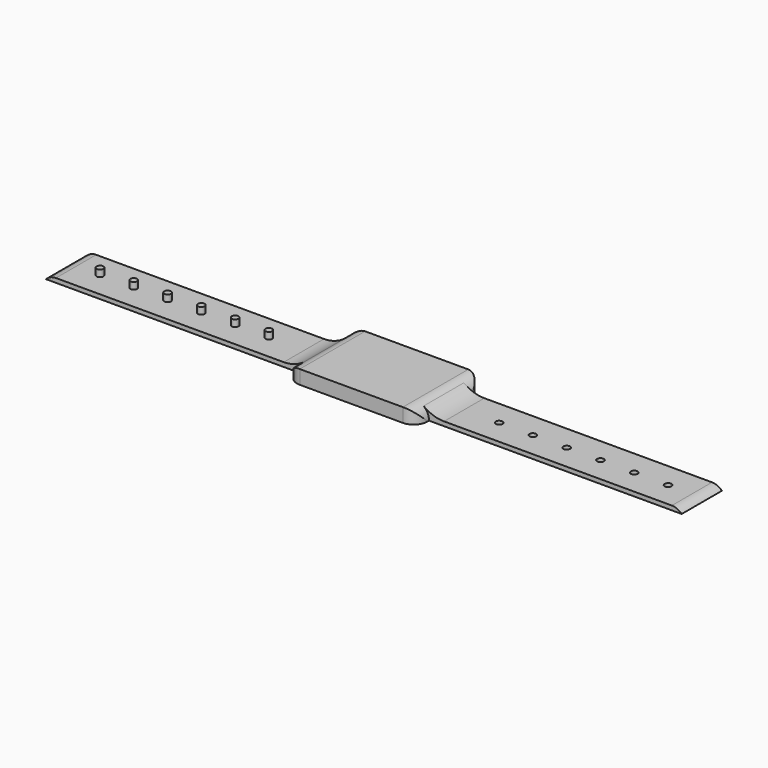
from build123d import *

# Parameters (mm, degrees)
F0_W         = 95.0192604214
F0_H         = 18.9093053341
F1_DEPTH     = 1.6002
F2_R         = 1.27
F3_DEPTH     = 25.4
F4_R         = 1.27
F5_DEPTH     = 2.54
F6_W         = 48.927821219
F6_H         = 30.7276230305
F7_DEPTH     = 3.6195
F8_T1_DEPTH  = 30.6197
F8_T6_DEPTH  = 56.1276230305
F8_T12_DEPTH = 56.1276230305
F8_T18_DEPTH = 56.1276230305
F8_T25_DEPTH = 56.1276230305
F8_T31_DEPTH = 56.1276230305
F8_T37_DEPTH = 56.1276230305
F8_T43_DEPTH = 56.1276230305
F8_T49_DEPTH = 56.1276230305
F8_T56_DEPTH = 56.1276230305
F8_T62_DEPTH = 56.1276230305
F9_T1_DEPTH  = 37.4142992276
F10_R        = 12.7


# Not quite as in the source:
# - a fillet or chamfer that OpenCascade refuses, or shapes differently, is made with other operations: its cross-section is extruded or revolved along the edge and cut away or added


with BuildPart() as f1:
    # F0 (on Top) → F1 (new body)
    with BuildSketch(Plane.XY):
        Polygon((-24.4639106095, -15.3638115153), (24.4639106095, -15.3638115153), (24.4639106095, -9.454652667), (24.4639106095, 9.454652667), (24.4639106095, 15.3638115153), (-24.4639106095, 15.3638115153), (-24.4639106095, 9.454652667), (-24.4639106095, -9.454652667), align=None)
        with Locations((71.9735408202, 0)):
            Rectangle(F0_W, F0_H)
        with Locations((-71.9735408202, 0)):
            Rectangle(F0_W, F0_H)
    extrude(amount=F1_DEPTH)

    # F2 (on face) → F3 (cut)
    with BuildSketch(Plane.XY.offset(1.6002)):
        with Locations((106.7831710309, 0)):
            Circle(F2_R)
        with Locations((94.0831710309, 0)):
            Circle(F2_R)
        with Locations((81.3831710309, 0)):
            Circle(F2_R)
        with Locations((68.6831710309, 0)):
            Circle(F2_R)
        with Locations((55.9831710309, 0)):
            Circle(F2_R)
        with Locations((43.2831710309, 0)):
            Circle(F2_R)
    extrude(amount=-F3_DEPTH, mode=Mode.SUBTRACT)

    # F4 (on face) → F5 (join)
    with BuildSketch(Plane.XY.offset(1.6002)):
        with Locations((-106.7719441229, 0)):
            Circle(F4_R)
        with Locations((-94.0719441229, 0)):
            Circle(F4_R)
        with Locations((-81.3719441229, 0)):
            Circle(F4_R)
        with Locations((-68.6719441229, 0)):
            Circle(F4_R)
        with Locations((-55.9719441229, 0)):
            Circle(F4_R)
        with Locations((-43.2719441229, 0)):
            Circle(F4_R)
    extrude(amount=F5_DEPTH)

    # F6 (on face) → F7 (join)
    with BuildSketch(Plane.XY.offset(1.6002)):
        Rectangle(F6_W, F6_H)
    extrude(amount=F7_DEPTH)

    # F8: fillet of radius 5.08 on 6 edges, made by hand

    # F8_s2 → F8_t1 (cut)
    with BuildSketch(Plane.XY.offset(-12.7)):
        with BuildLine():
            ThreePointArc((-19.3839106095, 15.3638115153), (-22.9760130579, 13.8759139637), (-24.4639106095, 10.2838115153))
            Line((-24.4639106095, 10.2838115153), (-24.4639106095, 15.3638115153))
            Line((-24.4639106095, 15.3638115153), (-19.3839106095, 15.3638115153))
        make_face()
        with BuildLine():
            ThreePointArc((-19.3839106095, -15.3638115153), (-22.9760130579, -13.8759139637), (-24.4639106095, -10.2838115153))
            Line((-24.4639106095, -10.2838115153), (-24.4639106095, -15.3638115153))
            Line((-24.4639106095, -15.3638115153), (-19.3839106095, -15.3638115153))
        make_face()
        with BuildLine():
            ThreePointArc((19.3839106095, -15.3638115153), (22.9760130579, -13.8759139637), (24.4639106095, -10.2838115153))
            Line((24.4639106095, -10.2838115153), (24.4639106095, -15.3638115153))
            Line((24.4639106095, -15.3638115153), (19.3839106095, -15.3638115153))
        make_face()
        with BuildLine():
            ThreePointArc((19.3839106095, 15.3638115153), (22.9760130579, 13.8759139637), (24.4639106095, 10.2838115153))
            Line((24.4639106095, 10.2838115153), (24.4639106095, 15.3638115153))
            Line((24.4639106095, 15.3638115153), (19.3839106095, 15.3638115153))
        make_face()
    extrude(amount=F8_T1_DEPTH, mode=Mode.SUBTRACT)


with BuildPart() as f8_tool4:
    # F8_s5 → F8_t6 (new body)
    with BuildSketch(Plane.XZ.offset(28.0638115153)):
        with BuildLine():
            ThreePointArc((24.4639106095, 0.1397), (22.9760130579, 3.7318024484), (19.3839106095, 5.2197))
            Line((19.3839106095, 5.2197), (24.4639106095, 5.2197))
            Line((24.4639106095, 5.2197), (24.4639106095, 0.1397))
        make_face()
    extrude(amount=-F8_T6_DEPTH)

    split(bisect_by=Plane.XY.offset(1.6002), keep=Keep.BOTTOM)

    split(bisect_by=Plane.XZ.offset(9.454652667), keep=Keep.TOP)


with BuildPart() as f1_1:
    add(f1.part)

    # F8_t3: cut F8_tool4
    add(f8_tool4.part, mode=Mode.SUBTRACT)


with BuildPart() as f8_tool10:
    # F8_s11 → F8_t12 (new body)
    with BuildSketch(Plane.XZ.offset(28.0638115153)):
        with BuildLine():
            ThreePointArc((24.4639106095, 0.1397), (22.9760130579, 3.7318024484), (19.3839106095, 5.2197))
            Line((19.3839106095, 5.2197), (24.4639106095, 5.2197))
            Line((24.4639106095, 5.2197), (24.4639106095, 0.1397))
        make_face()
    extrude(amount=-F8_T12_DEPTH)

    split(bisect_by=Plane.XY.offset(1.6002), keep=Keep.TOP)

    split(bisect_by=Plane.XZ.offset(9.454652667), keep=Keep.TOP)


with BuildPart() as f1_2:
    add(f1_1.part)

    # F8_t9: cut F8_tool10
    add(f8_tool10.part, mode=Mode.SUBTRACT)


with BuildPart() as f8_tool16:
    # F8_s17 → F8_t18 (new body)
    with BuildSketch(Plane.XZ.offset(28.0638115153)):
        with BuildLine():
            ThreePointArc((24.4639106095, 0.1397), (22.9760130579, 3.7318024484), (19.3839106095, 5.2197))
            Line((19.3839106095, 5.2197), (24.4639106095, 5.2197))
            Line((24.4639106095, 5.2197), (24.4639106095, 0.1397))
        make_face()
    extrude(amount=-F8_T18_DEPTH)

    split(bisect_by=Plane.XY.offset(1.6002), keep=Keep.TOP)

    split(bisect_by=Plane.XZ.offset(-9.454652667), keep=Keep.TOP)

    split(bisect_by=Plane.XZ.offset(9.454652667), keep=Keep.BOTTOM)


with BuildPart() as f1_3:
    add(f1_2.part)

    # F8_t15: cut F8_tool16
    add(f8_tool16.part, mode=Mode.SUBTRACT)


with BuildPart() as f8_tool23:
    # F8_s24 → F8_t25 (new body)
    with BuildSketch(Plane.XZ.offset(28.0638115153)):
        with BuildLine():
            ThreePointArc((24.4639106095, 0.1397), (22.9760130579, 3.7318024484), (19.3839106095, 5.2197))
            Line((19.3839106095, 5.2197), (24.4639106095, 5.2197))
            Line((24.4639106095, 5.2197), (24.4639106095, 0.1397))
        make_face()
    extrude(amount=-F8_T25_DEPTH)

    split(bisect_by=Plane.XY.offset(1.6002), keep=Keep.BOTTOM)

    split(bisect_by=Plane.XZ.offset(-9.454652667), keep=Keep.BOTTOM)


with BuildPart() as f1_4:
    add(f1_3.part)

    # F8_t22: cut F8_tool23
    add(f8_tool23.part, mode=Mode.SUBTRACT)


with BuildPart() as f8_tool29:
    # F8_s30 → F8_t31 (new body)
    with BuildSketch(Plane.XZ.offset(28.0638115153)):
        with BuildLine():
            ThreePointArc((24.4639106095, 0.1397), (22.9760130579, 3.7318024484), (19.3839106095, 5.2197))
            Line((19.3839106095, 5.2197), (24.4639106095, 5.2197))
            Line((24.4639106095, 5.2197), (24.4639106095, 0.1397))
        make_face()
    extrude(amount=-F8_T31_DEPTH)

    split(bisect_by=Plane.XY.offset(1.6002), keep=Keep.TOP)

    split(bisect_by=Plane.XZ.offset(-9.454652667), keep=Keep.BOTTOM)


with BuildPart() as f1_5:
    add(f1_4.part)

    # F8_t28: cut F8_tool29
    add(f8_tool29.part, mode=Mode.SUBTRACT)


with BuildPart() as f8_tool35:
    # F8_s36 → F8_t37 (new body)
    with BuildSketch(Plane.XZ.offset(-28.0638115153)):
        with BuildLine():
            ThreePointArc((-19.3839106095, 5.2197), (-22.9760130579, 3.7318024484), (-24.4639106095, 0.1397))
            Line((-24.4639106095, 0.1397), (-24.4639106095, 5.2197))
            Line((-24.4639106095, 5.2197), (-19.3839106095, 5.2197))
        make_face()
    extrude(amount=F8_T37_DEPTH)

    split(bisect_by=Plane.XZ.offset(-9.454652667), keep=Keep.BOTTOM)

    split(bisect_by=Plane.XY.offset(1.6002), keep=Keep.TOP)


with BuildPart() as f1_6:
    add(f1_5.part)

    # F8_t34: cut F8_tool35
    add(f8_tool35.part, mode=Mode.SUBTRACT)


with BuildPart() as f8_tool41:
    # F8_s42 → F8_t43 (new body)
    with BuildSketch(Plane.XZ.offset(-28.0638115153)):
        with BuildLine():
            ThreePointArc((-19.3839106095, 5.2197), (-22.9760130579, 3.7318024484), (-24.4639106095, 0.1397))
            Line((-24.4639106095, 0.1397), (-24.4639106095, 5.2197))
            Line((-24.4639106095, 5.2197), (-19.3839106095, 5.2197))
        make_face()
    extrude(amount=F8_T43_DEPTH)

    split(bisect_by=Plane.XZ.offset(-9.454652667), keep=Keep.BOTTOM)

    split(bisect_by=Plane.XY.offset(1.6002), keep=Keep.BOTTOM)


with BuildPart() as f1_7:
    add(f1_6.part)

    # F8_t40: cut F8_tool41
    add(f8_tool41.part, mode=Mode.SUBTRACT)


with BuildPart() as f8_tool47:
    # F8_s48 → F8_t49 (new body)
    with BuildSketch(Plane.XZ.offset(-28.0638115153)):
        with BuildLine():
            ThreePointArc((-19.3839106095, 5.2197), (-22.9760130579, 3.7318024484), (-24.4639106095, 0.1397))
            Line((-24.4639106095, 0.1397), (-24.4639106095, 5.2197))
            Line((-24.4639106095, 5.2197), (-19.3839106095, 5.2197))
        make_face()
    extrude(amount=F8_T49_DEPTH)

    split(bisect_by=Plane.XZ.offset(-9.454652667), keep=Keep.TOP)

    split(bisect_by=Plane.XY.offset(1.6002), keep=Keep.TOP)

    split(bisect_by=Plane.XZ.offset(9.454652667), keep=Keep.BOTTOM)


with BuildPart() as f1_8:
    add(f1_7.part)

    # F8_t46: cut F8_tool47
    add(f8_tool47.part, mode=Mode.SUBTRACT)


with BuildPart() as f8_tool54:
    # F8_s55 → F8_t56 (new body)
    with BuildSketch(Plane.XZ.offset(-28.0638115153)):
        with BuildLine():
            ThreePointArc((-19.3839106095, 5.2197), (-22.9760130579, 3.7318024484), (-24.4639106095, 0.1397))
            Line((-24.4639106095, 0.1397), (-24.4639106095, 5.2197))
            Line((-24.4639106095, 5.2197), (-19.3839106095, 5.2197))
        make_face()
    extrude(amount=F8_T56_DEPTH)

    split(bisect_by=Plane.XY.offset(1.6002), keep=Keep.TOP)

    split(bisect_by=Plane.XZ.offset(9.454652667), keep=Keep.TOP)


with BuildPart() as f1_9:
    add(f1_8.part)

    # F8_t53: cut F8_tool54
    add(f8_tool54.part, mode=Mode.SUBTRACT)


with BuildPart() as f8_tool60:
    # F8_s61 → F8_t62 (new body)
    with BuildSketch(Plane.XZ.offset(-28.0638115153)):
        with BuildLine():
            ThreePointArc((-19.3839106095, 5.2197), (-22.9760130579, 3.7318024484), (-24.4639106095, 0.1397))
            Line((-24.4639106095, 0.1397), (-24.4639106095, 5.2197))
            Line((-24.4639106095, 5.2197), (-19.3839106095, 5.2197))
        make_face()
    extrude(amount=F8_T62_DEPTH)

    split(bisect_by=Plane.XY.offset(1.6002), keep=Keep.BOTTOM)

    split(bisect_by=Plane.XZ.offset(9.454652667), keep=Keep.TOP)


with BuildPart() as f1_10:
    add(f1_9.part)

    # F8_t59: cut F8_tool60
    add(f8_tool60.part, mode=Mode.SUBTRACT)

    # F9: fillet of radius 5.08 on 2 edges, made by hand

    # F9_s2 → F9_t1 (cut)
    with BuildSketch(Plane.XZ.offset(-18.7071496138)):
        with BuildLine():
            ThreePointArc((115.7821722522, 1.6002), (117.7982347512, 1.1830201767), (119.4831710309, 0))
            Line((119.4831710309, 0), (119.4831710309, 1.6002))
            Line((119.4831710309, 1.6002), (115.7821722522, 1.6002))
        make_face()
        with BuildLine():
            ThreePointArc((-119.4831710309, 0), (-117.7982347512, 1.1830201767), (-115.7821722522, 1.6002))
            Line((-115.7821722522, 1.6002), (-119.4831710309, 1.6002))
            Line((-119.4831710309, 1.6002), (-119.4831710309, 0))
        make_face()
    extrude(amount=F9_T1_DEPTH, mode=Mode.SUBTRACT)

    # F10
    f10_edges = [f1_10.edges().sort_by_distance(p)[0] for p in [
        (24.249436, 0, 1.6002),
        (-24.249436, 0, 1.6002),
    ]]
    fillet(f10_edges, radius=F10_R)


solid = f1_10.part
